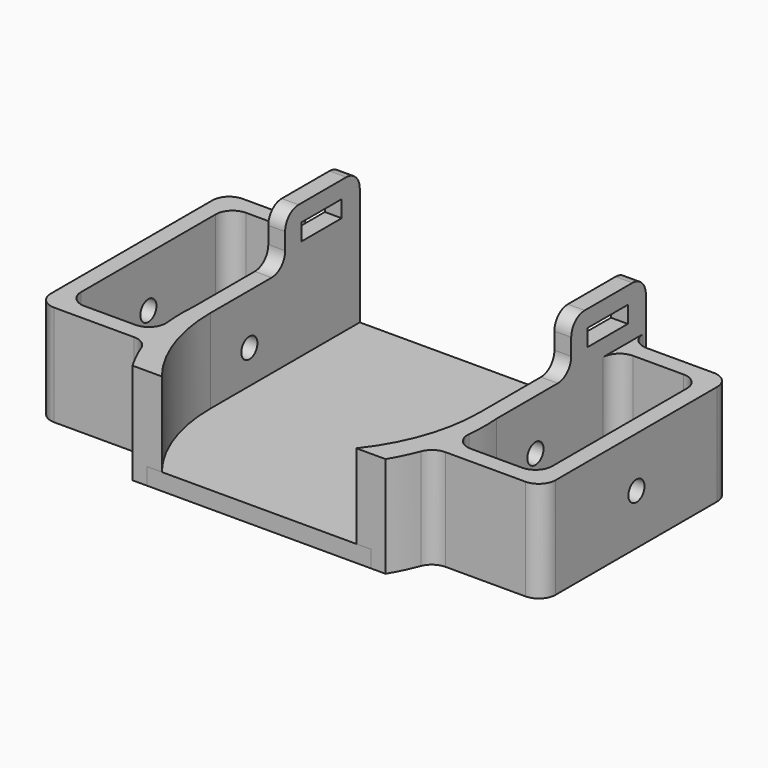
from build123d import *

# Parameters (mm, degrees)
F1_DEPTH  = 30
F3_DEPTH  = 5
F4_R      = 3
F5_DEPTH  = 35
F6_R      = 3
F7_DEPTH  = 35
F9_W      = 27.7209319142
F9_H      = 15
F9_W_2    = 15
F9_H_2    = 5
F10_DEPTH = 5
F11_R     = 5
F12_R     = 5
F13_R     = 5
F13_2_R   = 5
F14_R     = 5
F15_W     = 27.7209319142
F15_H     = 15
F15_W_2   = 15
F15_H_2   = 5
F16_DEPTH = 5
F17_R     = 5


with BuildPart() as f1:
    # F0 (on Top) → F1 (new body)
    with BuildSketch(Plane.XY):
        with BuildLine():
            Line((-45, 44.4425949542), (-45, 0))
            ThreePointArc((-45, 0), (-45.066266446, -7.8147796829), (-44.0046991035, -15.5574050458))
            ThreePointArc((-44.0046991035, -15.5574050458), (-43.4089049923, -18.0730910814), (-42.6934813561, -20.5574050458))
            ThreePointArc((-42.6934813561, -20.5574050458), (-40.475443237, -26.4101305765), (-37.5955815851, -31.9671519101))
            Line((-37.5955815851, -31.9671519101), (-28.8889932035, -31.9671519101))
            ThreePointArc((-28.8889932035, -31.9671519101), (-37.1430686541, -16.9215341597), (-40, 0))
            Line((-40, 0), (-40, 55.4418638284))
            Line((-40, 55.4418638284), (-45, 55.4418638284))
            Line((-45, 55.4418638284), (-45, 49.4425949542))
            Line((-45, 49.4425949542), (-45, 44.4425949542))
        make_face()
        with BuildLine():
            ThreePointArc((-42.6934813561, -20.5574050458), (-43.4089049923, -18.0730910814), (-44.0046991035, -15.5574050458))
            Line((-44.0046991035, -15.5574050458), (-70, -15.5574050458))
            Line((-70, -15.5574050458), (-70, 44.4425949542))
            Line((-70, 44.4425949542), (-45, 44.4425949542))
            Line((-45, 44.4425949542), (-45, 49.4425949542))
            Line((-45, 49.4425949542), (-75, 49.4425949542))
            Line((-75, 49.4425949542), (-75, -20.5574050458))
            Line((-75, -20.5574050458), (-42.6934813561, -20.5574050458))
        make_face()
    extrude(amount=F1_DEPTH)

    # F6 (on face) → F7 (cut)
    with BuildSketch(Plane(origin=(-75, 0, 0), x_dir=(0, -1, 0), z_dir=(-1, 0, 0))):
        with Locations((-14.4425949542, 15)):
            Circle(F6_R)
    extrude(amount=-F7_DEPTH, mode=Mode.SUBTRACT)

    # F9 (on face) → F10 (join)
    with BuildSketch(Plane(origin=(-45, 0, 0), x_dir=(0, -1, 0), z_dir=(-1, 0, 0))):
        with Locations((-41.5813978713, 37.5)):
            Rectangle(F9_W, F9_H)
        with Locations((-41.235268414, 37.4656194448)):
            Rectangle(F9_W_2, F9_H_2, mode=Mode.SUBTRACT)
    extrude(amount=-F10_DEPTH)

    # F11
    f11_edges = [f1.edges().sort_by_distance(p)[0] for p in [
        (-75, 49.442595, 15),
        (-75, -20.557405, 15),
    ]]
    fillet(f11_edges, radius=F11_R)

    # F13
    f13_edges = [f1.edges().sort_by_distance(p)[0] for p in [
        (-70, 44.442595, 15),
        (-70, -15.557405, 15),
        (-45, 44.442595, 15),
        (-44.004699, -15.557405, 15),
        (-42.693481, -20.557405, 15),
        (-45, 49.442595, 15),
        (-42.5, 27.720932, 30),
    ]]
    fillet(f13_edges, radius=F13_R)

    # F14
    f14_edges = [f1.edges().sort_by_distance(p)[0] for p in [
        (-42.5, 55.441864, 45),
        (-42.5, 27.720932, 45),
    ]]
    fillet(f14_edges, radius=F14_R)


with BuildPart() as f1b:
    # F0 (on Top) → F1, piece 2 (new body)
    with BuildSketch(Plane.XY):
        with BuildLine():
            ThreePointArc((44.0046991035, -15.5574050458), (45.066266446, -7.8147796829), (45, 0))
            Line((45, 0), (45, 44.4425949542))
            Line((45, 44.4425949542), (45, 49.4425949542))
            Line((45, 49.4425949542), (45, 55.4418638284))
            Line((45, 55.4418638284), (40, 55.4418638284))
            Line((40, 55.4418638284), (40, 0))
            ThreePointArc((40, 0), (37.1430686541, -16.9215341597), (28.8889932035, -31.9671519101))
            Line((28.8889932035, -31.9671519101), (37.5955815851, -31.9671519101))
            ThreePointArc((37.5955815851, -31.9671519101), (40.475443237, -26.4101305765), (42.6934813561, -20.5574050458))
            ThreePointArc((42.6934813561, -20.5574050458), (43.4089049923, -18.0730910814), (44.0046991035, -15.5574050458))
        make_face()
        with BuildLine():
            Line((45, 49.4425949542), (45, 44.4425949542))
            Line((45, 44.4425949542), (70, 44.4425949542))
            Line((70, 44.4425949542), (70, -15.5574050458))
            Line((70, -15.5574050458), (44.0046991035, -15.5574050458))
            ThreePointArc((44.0046991035, -15.5574050458), (43.4089049923, -18.0730910814), (42.6934813561, -20.5574050458))
            Line((42.6934813561, -20.5574050458), (75, -20.5574050458))
            Line((75, -20.5574050458), (75, 49.4425949542))
            Line((75, 49.4425949542), (45, 49.4425949542))
        make_face()
    extrude(amount=F1_DEPTH)

    # F4 (on face) → F5 (cut)
    with BuildSketch(Plane.YZ.offset(75)):
        with Locations((14.4425949542, 15)):
            Circle(F4_R)
    extrude(amount=-F5_DEPTH, mode=Mode.SUBTRACT)

    # F12
    f12_edges = [f1b.edges().sort_by_distance(p)[0] for p in [
        (75, -20.557405, 15),
        (75, 49.442595, 15),
    ]]
    fillet(f12_edges, radius=F12_R)

    # F13#2
    f13_2_edges = [f1b.edges().sort_by_distance(p)[0] for p in [
        (70, 44.442595, 15),
        (70, -15.557405, 15),
        (45, 44.442595, 15),
        (44.004699, -15.557405, 15),
        (42.693481, -20.557405, 15),
        (45, 49.442595, 15),
    ]]
    fillet(f13_2_edges, radius=F13_2_R)

    # F15 (on face) → F16 (join)
    with BuildSketch(Plane.YZ.offset(45)):
        with Locations((41.5813978713, 37.5)):
            Rectangle(F15_W, F15_H)
        with Locations((41.235268414, 37.4656194448)):
            Rectangle(F15_W_2, F15_H_2, mode=Mode.SUBTRACT)
    extrude(amount=-F16_DEPTH)

    # F17
    f17_edges = [f1b.edges().sort_by_distance(p)[0] for p in [
        (42.5, 55.441864, 45),
        (42.5, 27.720932, 45),
        (42.5, 27.720932, 30),
    ]]
    fillet(f17_edges, radius=F17_R)


with BuildPart() as f3:
    # F2 (on face) → F3 (new body)
    with BuildSketch(Plane(origin=(0, 0, 0), x_dir=(1, 0, 0), z_dir=(0, 0, -1))):
        Polygon((-42.5, 0), (-42.5, -55.4418638284), (0, -55.4418638284), (0, 31.9671519101), (-33.2422873943, 31.9671519101), align=None)
        Polygon((0, 31.9671519101), (0, -55.4418638284), (42.5, -55.4418638284), (42.5, 0), (33.2422873943, 31.9671519101), align=None)
    extrude(amount=-F3_DEPTH)


solid = Compound([f1.part, f1b.part, f3.part])
